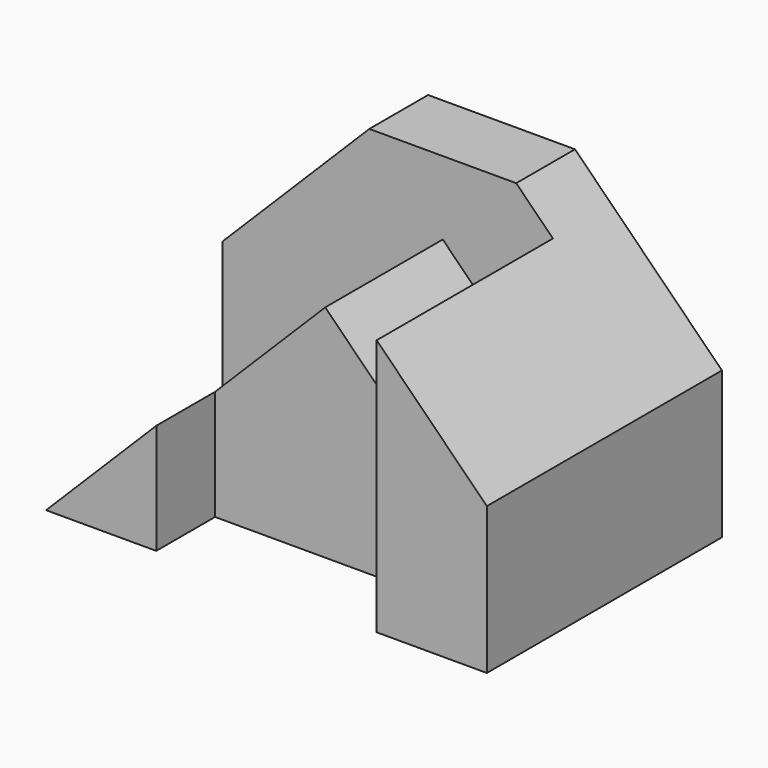
from build123d import *

# Parameters (mm, degrees)
F0_W     = 19.05
F0_H     = 12.7
F0_W_2   = 31.75
F1_DEPTH = 50.8
F3_DEPTH = 50.801
F7_DEPTH = 38.1
F8_DEPTH = 25.4


# Not quite as in the source:
# - a feature names something its author has since deleted; it is built from what else it names


with BuildPart() as f1:
    # F0 (on Top) → F1 (new body)
    with BuildSketch(Plane.XY):
        with Locations((-28.575, 6.35)):
            Rectangle(F0_W, F0_H)
        with Locations((22.225, 6.35)):
            Rectangle(F0_W_2, F0_H)
        Polygon((-19.05, 0), (0, 0), (6.35, 0), (6.35, 12.7), (-19.05, 12.7), align=None)
        Polygon((6.35, 0), (0, 0), (38.1, -38.1), (38.1, 0), align=None)
        Polygon((-38.1, -38.1), (0, 0), (-19.05, 0), (-38.1, 0), align=None)
        Polygon((38.1, -38.1), (0, 0), (-38.1, -38.1), (-19.05, -38.1), (-19.05, -25.4), (19.05, -25.4), (19.05, -38.1), align=None)
    extrude(amount=F1_DEPTH)

    # F2 (on face) → F3 (cut, through all)
    with BuildSketch(Plane(origin=(0, 12.7, 0), x_dir=(-1, 0, 0), z_dir=(0, 1, 0))):
        Polygon((-38.1, 50.8), (-38.1, 25.4), (-12.7, 50.8), align=None)
        Polygon((38.1, 50.8), (12.7, 50.8), (38.1, 25.4), align=None)
    extrude(amount=-F3_DEPTH, mode=Mode.SUBTRACT)

    # F4 (on face) → F7 (cut)
    with BuildSketch(Plane.XZ.offset(38.1)):
        Polygon((-38.1, 25.4), (-38.1, 0), (-19.05, 19.05), (-19.05, 44.45), align=None)
    extrude(amount=-F7_DEPTH, mode=Mode.SUBTRACT)

    # F5 (on face) → F8 (cut)
    with BuildSketch(Plane.XZ.offset(25.4)):
        Polygon((-19.05, 44.45), (-19.05, 19.05), (0, 38.1), (19.05, 19.05), (19.05, 44.45), (12.7, 50.8), (-12.7, 50.8), align=None)
    extrude(amount=-F8_DEPTH, mode=Mode.SUBTRACT)


solid = f1.part
